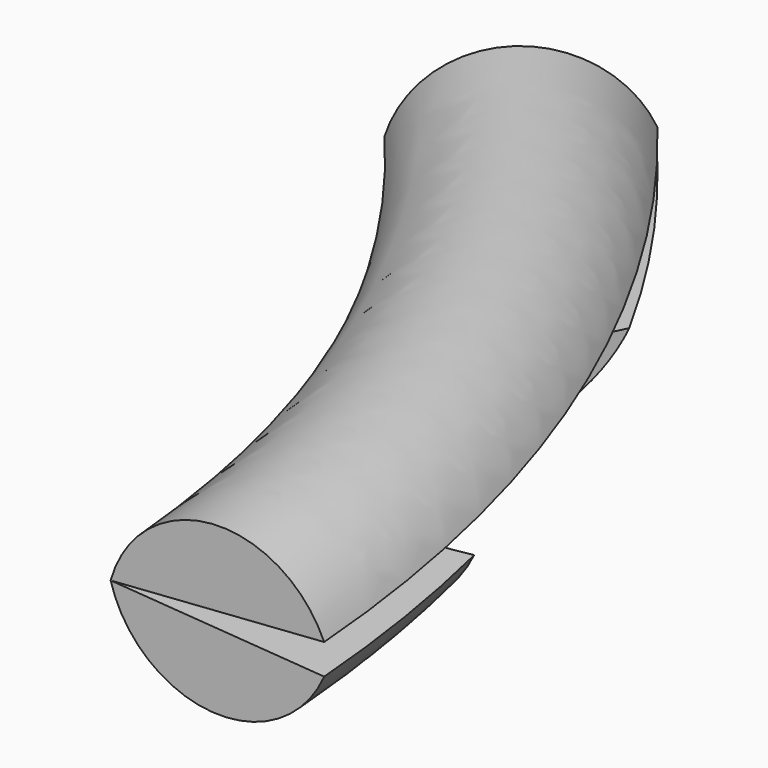
from build123d import *

# Parameters (mm, degrees)
F5_DEPTH = 19.685


with BuildPart() as f2:
    # F2: sweep along a path in F1
    with BuildLine(Plane.XY) as f2_path:
        ThreePointArc((2.5794103276, 0), (-13.1552361752, 65.0705018825), (-47.7892048657, 122.361317277))
    # F0 (on Front) → F2 (sweep)
    with BuildSketch(Plane.XZ):
        with BuildLine():
            Line((-13.9575442299, 0), (19.5197295398, 2.3856847547))
            ThreePointArc((19.5197295398, 2.3856847547), (1.9408124217, 12.9841284446), (-13.9575442299, 0))
        make_face()
    sweep(path=f2_path.line)


with BuildPart() as f3_1:
    # F3: instance of F2
    add(f2.part.mirror(Plane.XY))

    # F4 (on Top) → F5 (cut, symmetric)
    with BuildSketch(Plane.XY):
        with BuildLine():
            ThreePointArc((41.7517051101, 74.454382062), (28.6847679393, 100.99919665), (2.3437023629, 114.472143352))
            ThreePointArc((2.3437023629, 114.472143352), (-13.8641041279, 75.7926532577), (-5.4263374768, 34.7122438252))
            ThreePointArc((-5.4263374768, 34.7122438252), (26.9606147491, 44.1392558641), (41.7517051101, 74.454382062))
        make_face()
    extrude(amount=F5_DEPTH, both=True, mode=Mode.SUBTRACT)


solid = Compound([f2.part, f3_1.part])
